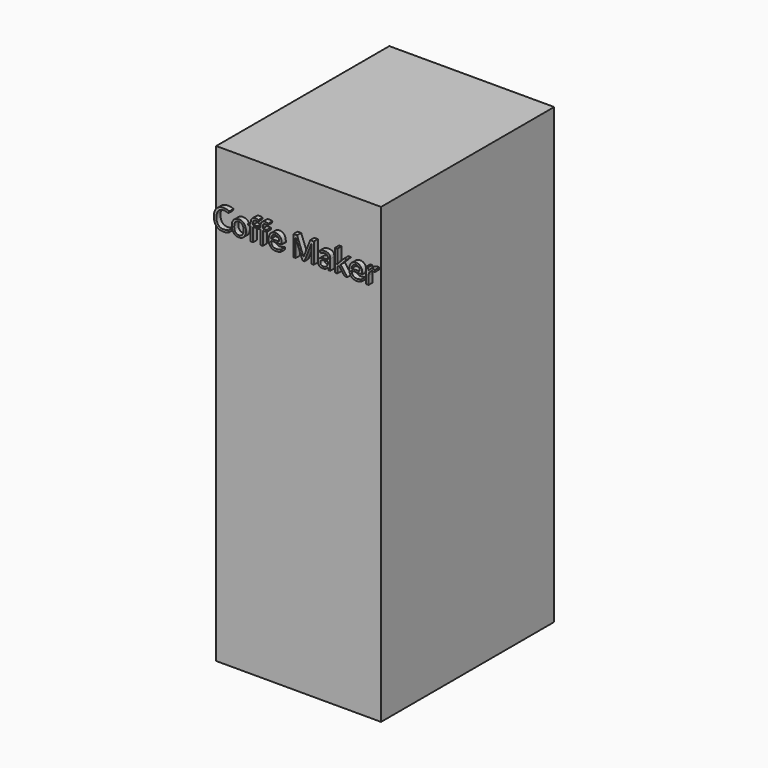
from build123d import *

# Parameters (mm, degrees)
F0_W         = 203.2
F0_H         = 558.8
F1_DEPTH     = 266.7
F3_TEXT_SIZE = 35.4141592655
F4_DEPTH     = 6.35


# Not quite as in the source:
# - Text() gives the source's letters only with a copy of the font that has no kerning and outlines rounded to 1/6400 em; it was checked with that copy


with BuildPart() as f1:
    # F0 (on Front) → F1 (new body)
    with BuildSketch(Plane.XZ):
        with Locations((101.6, 279.4)):
            Rectangle(F0_W, F0_H)
    extrude(amount=F1_DEPTH)

    # F3 (on face) → F4 (join)
    with BuildSketch(Plane.XZ.offset(266.7)):
        with Locations((0, 473.2774353105)):
            Text('Coffe Maker', F3_TEXT_SIZE, font='Open Sans', text_align=(TextAlign.LEFT, TextAlign.BOTTOM))
    extrude(amount=F4_DEPTH)


solid = f1.part
